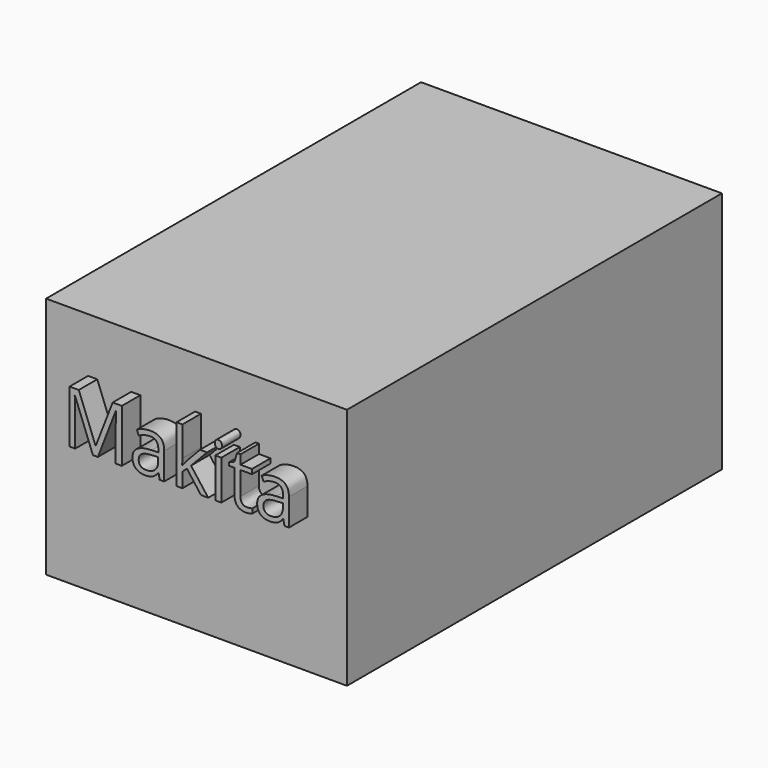
from build123d import *

# Parameters (mm, degrees)
F0_W         = 330.2
F0_H         = 266.7
F1_DEPTH     = 514.35
F2_TEXT_SIZE = 81.1582626061
F3_DEPTH     = 25.4


# Not quite as in the source:
# - Text() gives the source's letters only with a copy of the font that has no kerning and outlines rounded to 1/6400 em; it was checked with that copy


with BuildPart() as f1:
    # F0 (on Front) → F1 (new body)
    with BuildSketch(Plane.XZ):
        Rectangle(F0_W, F0_H)
    extrude(amount=F1_DEPTH)

    # F2 (on face) → F3 (join)
    with BuildSketch(Plane.XZ.offset(514.35)):
        with Locations((-127, 15.7368079125)):
            Text('Makita', F2_TEXT_SIZE, font='Open Sans', text_align=(TextAlign.LEFT, TextAlign.BOTTOM))
    extrude(amount=F3_DEPTH)


solid = f1.part
